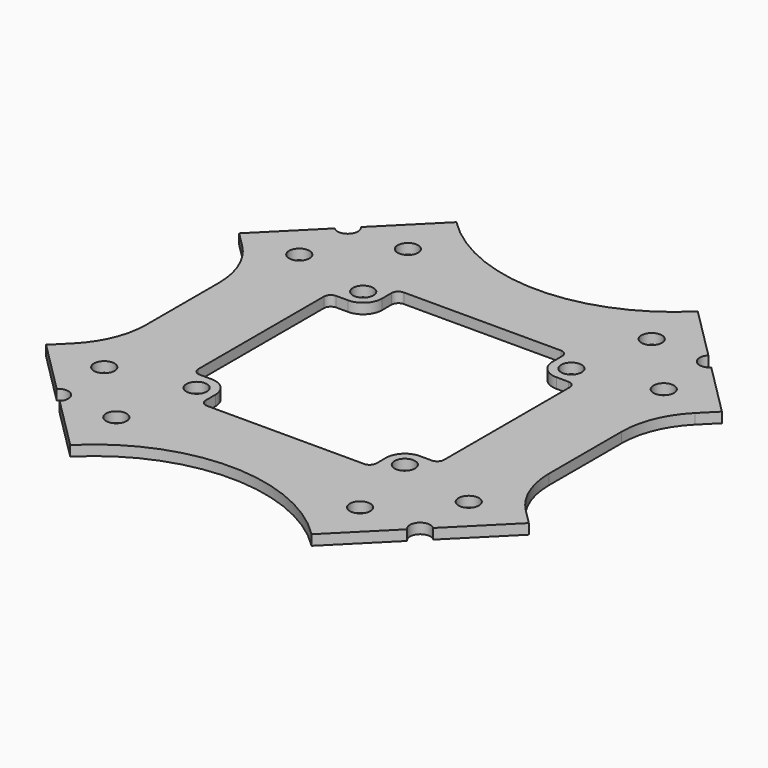
from build123d import *

# Parameters (mm, degrees)
F0_R     = 1.5
F1_DEPTH = 1.5


# Not quite as in the source:
# - ends of sketch curves that miss each other by under 0.0002 mm in the source are joined


with BuildPart() as f1:
    # F0 (on Top) → F1 (new body)
    with BuildSketch(Plane.XY):
        with BuildLine():
            Line((-29.5, 6.644661), (-29.5, 0))
            Line((-29.5, 0), (-29.5, -6.644661))
            ThreePointArc((-29.5, -6.644661), (-30.4515057083, -11.4282035779), (-33.1611647352, -15.4834952648))
            Line((-33.1611647352, -15.4834952648), (-35.355339, -17.677669))
            Line((-35.355339, -17.677669), (-27.577165, -25.455844))
            ThreePointArc((-27.577165, -25.455844), (-25.4558450782, -25.4558435782), (-25.4558443282, -27.5771636718))
            Line((-25.4558443282, -27.5771636718), (-17.67767, -35.355339))
            ThreePointArc((-17.67767, -35.355339), (-3.536e-07, -28.033008), (17.6776695297, -35.3553384703))
            Line((17.6776695297, -35.3553384703), (25.455844, -27.577164))
            ThreePointArc((25.455844, -27.577164), (25.4558438282, -25.4558438282), (27.5771641718, -25.4558438282))
            Line((27.5771641718, -25.4558438282), (35.355339, -17.677669))
            Line((35.355339, -17.677669), (33.161165, -15.483495))
            ThreePointArc((33.161165, -15.483495), (30.4515057083, -11.4282035779), (29.5, -6.644661))
            Line((29.5, -6.644661), (29.5, 0))
            Line((29.5, 0), (29.5, 6.644661))
            ThreePointArc((29.5, 6.644661), (30.4515058436, 11.4282039046), (33.1611652352, 15.4834957648))
            Line((33.1611652352, 15.4834957648), (35.355339, 17.67767))
            Line((35.355339, 17.67767), (27.577164, 25.455844))
            ThreePointArc((27.577164, 25.455844), (25.4558435782, 25.4558450782), (25.4558438282, 27.5771651718))
            Line((25.4558438282, 27.5771651718), (17.677669, 35.355339))
            ThreePointArc((17.677669, 35.355339), (-3.536e-07, 28.033009), (-17.6776695297, 35.3553394703))
            Line((-17.6776695297, 35.3553394703), (-25.455844, 27.577165))
            ThreePointArc((-25.455844, 27.577165), (-25.4558448282, 25.4558448282), (-27.5771646718, 25.4558443282))
            Line((-27.5771646718, 25.4558443282), (-35.355339, 17.67767))
            Line((-35.355339, 17.67767), (-33.161165, 15.483496))
            ThreePointArc((-33.161165, 15.483496), (-30.4515058436, 11.4282039046), (-29.5, 6.644661))
        make_face()
        with Locations((-17.854446, -26.693281)):
            Circle(F0_R, mode=Mode.SUBTRACT)
        with Locations((-26.693281, -17.854446)):
            Circle(F0_R, mode=Mode.SUBTRACT)
        with Locations((-15.25, -15.25)):
            Circle(F0_R, mode=Mode.SUBTRACT)
        with Locations((17.854446, -26.693281)):
            Circle(F0_R, mode=Mode.SUBTRACT)
        with Locations((26.693281, -17.854446)):
            Circle(F0_R, mode=Mode.SUBTRACT)
        with Locations((15.25, -15.25)):
            Circle(F0_R, mode=Mode.SUBTRACT)
        with BuildLine():
            Line((11.5, -18), (-11.5, -18))
            ThreePointArc((-11.5, -18), (-12.2071067812, -17.7071067812), (-12.5, -17))
            Line((-12.5, -17), (-12.5, -15.25))
            ThreePointArc((-12.5, -15.25), (-13.3054563517, -13.3054563517), (-15.25, -12.5))
            Line((-15.25, -12.5), (-17, -12.5))
            ThreePointArc((-17, -12.5), (-17.7071067812, -12.2071067812), (-18, -11.5))
            Line((-18, -11.5), (-18, 11.5))
            ThreePointArc((-18, 11.5), (-17.7071067812, 12.2071067812), (-17, 12.5))
            Line((-17, 12.5), (-15.25, 12.5))
            ThreePointArc((-15.25, 12.5), (-13.3054563517, 13.3054563517), (-12.5, 15.25))
            Line((-12.5, 15.25), (-12.5, 17))
            ThreePointArc((-12.5, 17), (-12.2071067812, 17.7071067812), (-11.5, 18))
            Line((-11.5, 18), (11.5, 18))
            ThreePointArc((11.5, 18), (12.2071067812, 17.7071067812), (12.5, 17))
            Line((12.5, 17), (12.5, 15.25))
            ThreePointArc((12.5, 15.25), (13.3054563517, 13.3054563517), (15.25, 12.5))
            Line((15.25, 12.5), (17, 12.5))
            ThreePointArc((17, 12.5), (17.7071067812, 12.2071067812), (18, 11.5))
            Line((18, 11.5), (18, -11.5))
            ThreePointArc((18, -11.5), (17.7071067812, -12.2071067812), (17, -12.5))
            Line((17, -12.5), (15.25, -12.5))
            ThreePointArc((15.25, -12.5), (13.3054563517, -13.3054563517), (12.5, -15.25))
            Line((12.5, -15.25), (12.5, -17))
            ThreePointArc((12.5, -17), (12.2071067812, -17.7071067812), (11.5, -18))
        make_face(mode=Mode.SUBTRACT)
        with Locations((-15.25, 15.25)):
            Circle(F0_R, mode=Mode.SUBTRACT)
        with Locations((-26.693281, 17.854447)):
            Circle(F0_R, mode=Mode.SUBTRACT)
        with Locations((-17.854446, 26.693281)):
            Circle(F0_R, mode=Mode.SUBTRACT)
        with Locations((15.25, 15.25)):
            Circle(F0_R, mode=Mode.SUBTRACT)
        with Locations((26.693281, 17.854447)):
            Circle(F0_R, mode=Mode.SUBTRACT)
        with Locations((17.854446, 26.693281)):
            Circle(F0_R, mode=Mode.SUBTRACT)
    extrude(amount=F1_DEPTH)


solid = f1.part
